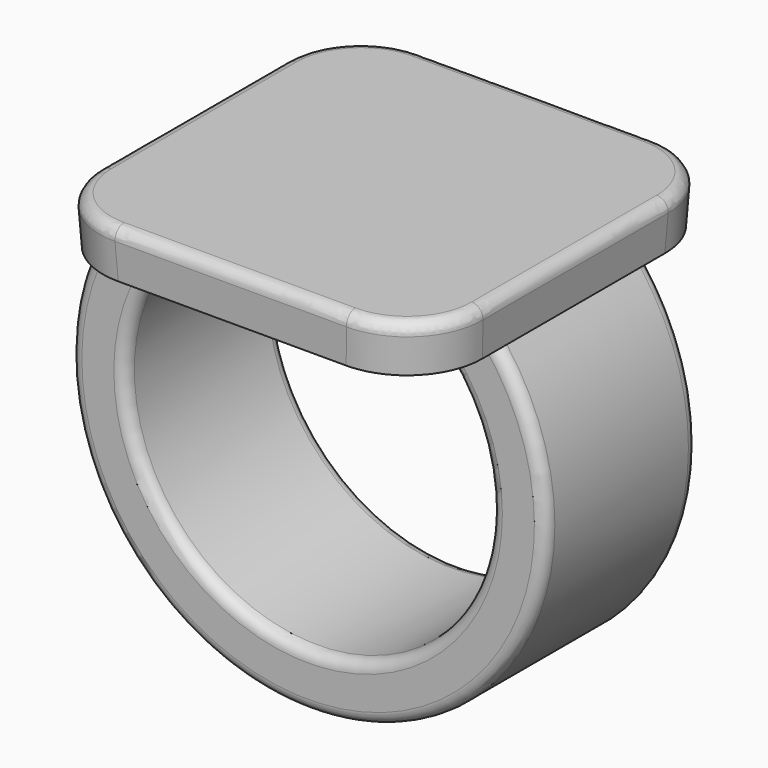
from build123d import *

# Parameters (mm, degrees)
F0_W          = 25.4
F0_H          = 25.4
F1_DEPTH      = 3.175
F1_TAPER      = -3
F3_W          = 5.08
F3_H          = 12.7
F6_DEPTH      = 6.35
F6_DEPTH_BACK = 6.35
F7_R          = 5.08
F8_R          = 0.762


# Not quite as in the source:
# - a feature of the source that left no trace in its solid (it failed there, or was rolled back) is left out


with BuildPart() as f1:
    # F0 (on Top) → F1 (new body)
    with BuildSketch(Plane.XY):
        Rectangle(F0_W, F0_H)
    extrude(amount=F1_DEPTH, taper=F1_TAPER)

    # F4: sweep along a path in F2
    with BuildLine(Plane.XZ) as f4_path:
        ThreePointArc((-10.16, 0), (0, -23.5582897328), (10.16, 0))
    # F3 (on face) → F4 (sweep)
    with BuildSketch(Plane(origin=(0, 0, 0), x_dir=(1, 0, 0), z_dir=(0, 0, -1))):
        with Locations((-10.16, 0)):
            Rectangle(F3_W, F3_H)
    sweep(path=f4_path.line)

    # F5 (on Front) → F6 (join, two sides)
    with BuildSketch(Plane.XZ) as f6_sk:
        with BuildLine():
            ThreePointArc((7.62, 0), (8.9072265211, -1.1822790439), (10.0130578512, -2.535746045))
            Line((10.0130578512, -2.535746045), (10.16, 0))
            Line((10.16, 0), (7.62, 0))
        make_face()
    extrude(amount=F6_DEPTH)
    extrude(f6_sk.sketch, amount=-F6_DEPTH_BACK)

    # F7
    f7_edges = [f1.edges().sort_by_distance(p)[0] for p in [
        (-12.783197, -12.783197, 1.5875),
        (12.783197, 12.783197, 1.5875),
        (12.783197, -12.783197, 1.5875),
        (-12.783197, 12.783197, 1.5875),
    ]]
    fillet(f7_edges, radius=F7_R)

    # F8
    f8_edges = [f1.edges().sort_by_distance(p)[0] for p in [
        (-1.743325, 6.35, -21.711017),
        (8.907227, 6.35, -1.182279),
        (-1.743325, -6.35, -21.711017),
        (0, 12.866395, 3.175),
        (11.381365, 11.381391, 3.175),
        (-11.381365, 11.381391, 3.175),
        (12.866395, 0, 3.175),
        (-12.866395, 0, 3.175),
        (11.381391, -11.381365, 3.175),
        (-11.381365, -11.381391, 3.175),
        (0, -12.866395, 3.175),
        (0, 6.35, -25.501344),
        (8.907227, -6.35, -1.182279),
        (0, -6.35, -25.501344),
    ]]
    fillet(f8_edges, radius=F8_R)


solid = f1.part
